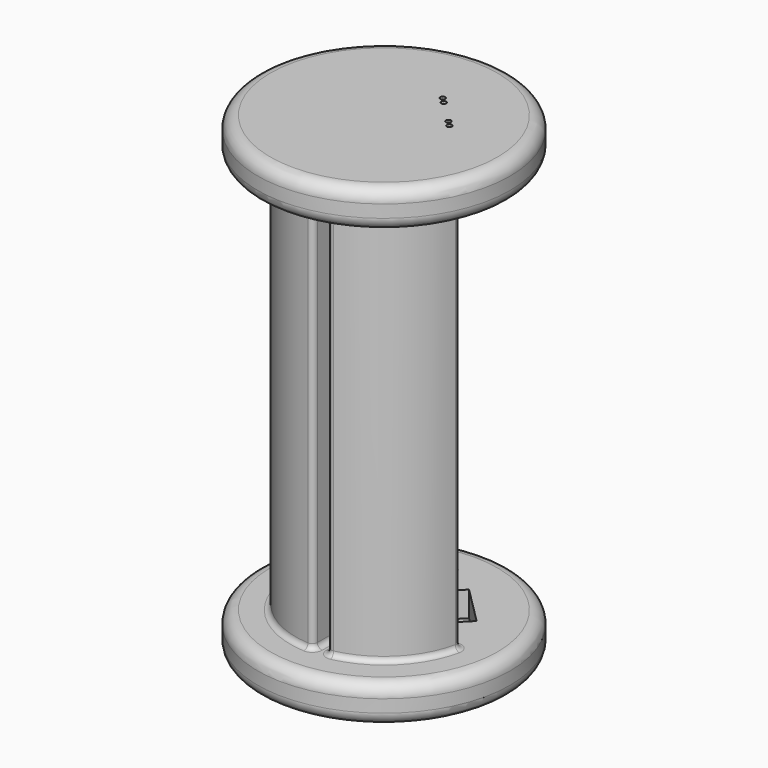
from build123d import *

# Parameters (mm, degrees)
F0_R      = 127
F1_DEPTH  = 38.1
F2_W      = 88.9
F2_H      = 399.9992
F3_ANGLE  = 278
F4_W      = 127
F4_H      = 38.1
F6_W      = 12.7
F6_H      = 399.9992
F7_DEPTH  = 1270
F8_W      = 12.7
F8_H      = 399.9992
F9_DEPTH  = 1270
F10_R     = 63.5
F11_DEPTH = 399.9992
F12_R     = 12.7
F13_R     = 12.7
F14_F1_R  = 5.08
F14_F2_R  = 5.08
F16_DEPTH = 25.4
F18_DEPTH = 38.101
F19_DEPTH = 38.101


with BuildPart() as f1:
    # F0 (on Top) → F1 (new body)
    with BuildSketch(Plane.XY):
        Circle(F0_R)
    extrude(amount=F1_DEPTH)

    # F2 (on Front) → F3 (revolve)
    with BuildSketch(Plane.XZ):
        with Locations((44.45, -199.9996)):
            Rectangle(F2_W, F2_H)
    revolve(axis=Axis((0, 0, -199.9996), (0, 0, -1)), revolution_arc=F3_ANGLE)

    # F4 (on Front) → F5 (revolve)
    with BuildSketch(Plane.XZ):
        with Locations((63.5, -419.0492)):
            Rectangle(F4_W, F4_H)
    revolve(axis=Axis((0, 0, -399.9992), (0, 0, 1)))

    # F6 (on Front) → F7 (cut, symmetric)
    with BuildSketch(Plane.XZ):
        with Locations((6.35, -199.9996)):
            Rectangle(F6_W, F6_H)
    extrude(amount=F7_DEPTH, both=True, mode=Mode.SUBTRACT)

    # F8 (on Right) → F9 (cut, symmetric)
    with BuildSketch(Plane.YZ):
        with Locations((-6.35, -199.9996)):
            Rectangle(F8_W, F8_H)
    extrude(amount=F9_DEPTH, both=True, mode=Mode.SUBTRACT)

    # F10 (on Top) → F11 (cut)
    with BuildSketch(Plane.XY):
        Circle(F10_R)
    extrude(amount=-F11_DEPTH, mode=Mode.SUBTRACT)

    # F12
    f12_edges = [f1.edges().sort_by_distance(p)[0] for p in [
        (127, 0, 19.05),
        (-127, 0, 0),
        (-127, 0, 38.1),
    ]]
    fillet(f12_edges, radius=F12_R)

    # F13
    f13_edges = [f1.edges().sort_by_distance(p)[0] for p in [
        (-127, 0, -438.0992),
        (127, 0, -419.0492),
        (-127, 0, -399.9992),
    ]]
    fillet(f13_edges, radius=F13_R)

    # F14: fillet of radius 5.08 on 18 edges, made by hand

    # F14_f1
    f14_f1_edges = [f1.edges().sort_by_distance(p)[0] for p in [
        (87.9881810245, -12.7, -199.9996),
        (12.7, -87.9881810245, -199.9996),
        (0, -88.9, -199.9996),
        (-87.9881810245, -12.7, -199.9996),
        (-88.9, 0, -199.9996),
        (0, 88.9, -199.9996),
    ]]
    fillet(f14_f1_edges, radius=F14_F1_R)

    # F14_f2
    f14_f2_edges = [f1.edges().sort_by_distance(p)[0] for p in [
        (62.8617928475, -62.8617928475, 0),
        (62.8617928475, -62.8617928475, -399.9992),
        (-57.8702669833, -67.4851257632, 0),
        (-57.8702669833, -67.4851257632, -399.9992),
        (-62.8617928475, 62.8617928475, 0),
        (-62.8617928475, 62.8617928475, -399.9992),
        (0, 73.5829594937, -399.9992),
        (-73.5829594937, 0, -399.9992),
        (0, -73.5829594937, -399.9992),
        (0, 73.5829594937, 0),
        (-73.5829594937, 0, 0),
        (0, -73.5829594937, 0),
        (-1.5984503624, -87.3652719201, 0),
        (-87.3652719201, 1.5984503624, 0),
        (-1.5984503624, 87.3652719201, 0),
        (-1.5984503624, -87.3652719201, -399.9992),
        (-87.3652719201, 1.5984503624, -399.9992),
        (-1.5984503624, 87.3652719201, -399.9992),
        (-85.8673133591, -14.5915587545, -399.9992),
        (-85.8673133591, -14.5915587545, 0),
        (85.8673133591, -14.5915587545, -399.9992),
        (14.5915587545, -85.8673133591, -399.9992),
        (85.8673133591, -14.5915587545, 0),
        (14.5915587545, -85.8673133591, 0),
    ]]
    fillet(f14_f2_edges, radius=F14_F2_R)

    # F15 (on face) → F16 (cut)
    with BuildSketch(Plane.XY.offset(-399.9992)):
        Polygon((30.6240873449, 68.7240873449), (20.32, 58.42), (58.42, 20.32), (68.7240873449, 30.6240873449), align=None)
    extrude(amount=-F16_DEPTH, mode=Mode.SUBTRACT)

    # F17 (on face) → F18 (cut, through all)
    with BuildSketch(Plane(origin=(0, 0, 0), x_dir=(1, 0, 0), z_dir=(0, 0, -1))):
        with BuildLine():
            ThreePointArc((21.6051478316, -47.8954906697), (24.373214974, -48.446093458), (25.9411990558, -46.0994394454))
            ThreePointArc((25.9411990558, -46.0994394454), (25.7478530684, -45.1274235272), (25.19725028, -44.3033882212))
            Line((25.19725028, -44.3033882212), (21.6051478316, -47.8954906697))
        make_face()
        with BuildLine():
            Line((21.6051478316, -47.8954906697), (25.19725028, -44.3033882212))
            ThreePointArc((25.19725028, -44.3033882212), (21.6051478316, -44.3033882212), (21.6051478316, -47.8954906697))
        make_face()
        with BuildLine():
            Line((47.8954906697, -21.6051478316), (44.3033882212, -25.19725028))
            ThreePointArc((44.3033882212, -25.19725028), (47.0714553637, -25.7478530684), (48.6394394454, -23.4011990558))
            ThreePointArc((48.6394394454, -23.4011990558), (48.446093458, -22.4291831376), (47.8954906697, -21.6051478316))
        make_face()
        with BuildLine():
            ThreePointArc((47.8954906697, -21.6051478316), (44.3033882212, -21.6051478316), (44.3033882212, -25.19725028))
            Line((44.3033882212, -25.19725028), (47.8954906697, -21.6051478316))
        make_face()
    extrude(amount=-F18_DEPTH, mode=Mode.SUBTRACT)

    # F17 (on face) → F19 (cut, through all)
    with BuildSketch(Plane(origin=(0, 0, 0), x_dir=(1, 0, 0), z_dir=(0, 0, -1))):
        with BuildLine():
            ThreePointArc((20.5530453832, -51.4875931181), (20.3596993958, -50.5155771999), (19.8090966074, -49.6915418939))
            Line((19.8090966074, -49.6915418939), (16.216994159, -53.2836443423))
            ThreePointArc((16.216994159, -53.2836443423), (18.9850613014, -53.8342471307), (20.5530453832, -51.4875931181))
        make_face()
        with BuildLine():
            Line((16.216994159, -53.2836443423), (19.8090966074, -49.6915418939))
            ThreePointArc((19.8090966074, -49.6915418939), (16.216994159, -49.6915418939), (16.216994159, -53.2836443423))
        make_face()
        with BuildLine():
            Line((53.2836443423, -16.216994159), (49.6915418939, -19.8090966074))
            ThreePointArc((49.6915418939, -19.8090966074), (52.4596090363, -20.3596993958), (54.0275931181, -18.0130453832))
            ThreePointArc((54.0275931181, -18.0130453832), (53.8342471307, -17.041029465), (53.2836443423, -16.216994159))
        make_face()
        with BuildLine():
            ThreePointArc((53.2836443423, -16.216994159), (49.6915418939, -16.216994159), (49.6915418939, -19.8090966074))
            Line((49.6915418939, -19.8090966074), (53.2836443423, -16.216994159))
        make_face()
    extrude(amount=-F19_DEPTH, mode=Mode.SUBTRACT)


solid = f1.part
